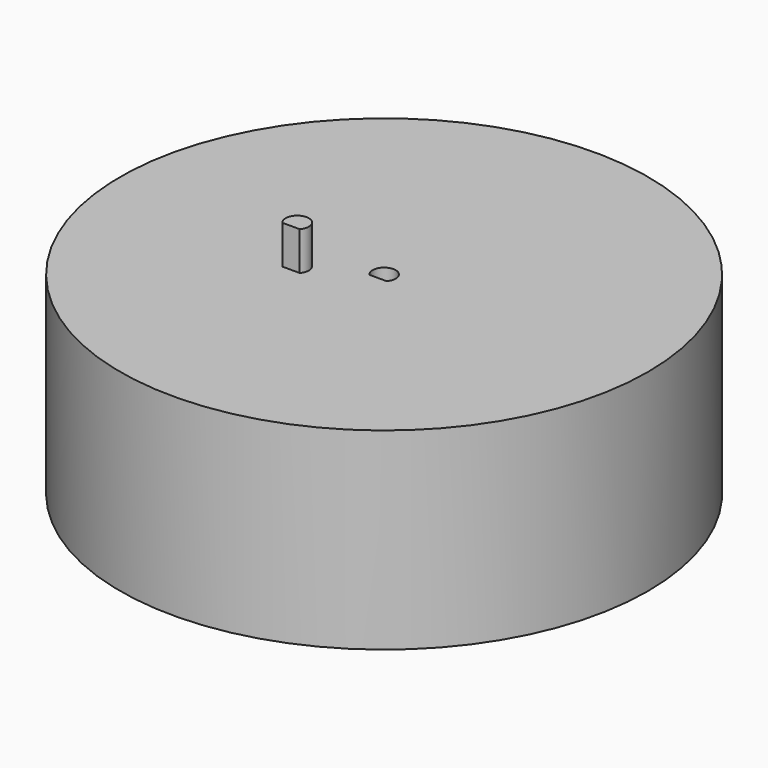
from build123d import *

# Parameters (mm, degrees)
F0_R     = 34.2051900743
F1_DEPTH = 25
F3_DEPTH = 10
F4_W     = 10
F4_H     = 7
F5_DEPTH = 20
F7_DEPTH = 10


with BuildPart() as f1:
    # F0 (on Top) → F1 (new body)
    with BuildSketch(Plane.XY):
        Circle(F0_R)
    extrude(amount=F1_DEPTH)

    # F2 (on face) → F3 (cut)
    with BuildSketch(Plane.XY.offset(25)):
        with BuildLine():
            Line((0, -1), (1.1180339887, -1))
            ThreePointArc((1.1180339887, -1), (0, 1.5), (-1.1180339887, -1))
            Line((-1.1180339887, -1), (0, -1))
        make_face()
    extrude(amount=-F3_DEPTH, mode=Mode.SUBTRACT)


with BuildPart() as f5:
    # F4 (on Top) → F5 (new body)
    with BuildSketch(Plane.XY):
        with Locations((-7.8889451153, -4.0067454018)):
            Rectangle(F4_W, F4_H)
        with BuildLine():
            Line((-12.8889451153, -0.5067454018), (-2.8889451153, -0.5067454018))
            ThreePointArc((-2.8889451153, -0.5067454018), (-7.8889451153, 2.2227708057), (-12.8889451153, -0.5067454018))
        make_face()
        with BuildLine():
            ThreePointArc((-12.8889451153, -7.5067454018), (-7.8889451153, -9.9842291943), (-2.8889451153, -7.5067454018))
            Line((-2.8889451153, -7.5067454018), (-12.8889451153, -7.5067454018))
        make_face()
    extrude(amount=F5_DEPTH)

    # F6 (on face) → F7 (join)
    with BuildSketch(Plane.XY.offset(20)):
        with BuildLine():
            Line((-7.9751741141, -5.0994232297), (-6.8571401254, -5.0994232297))
            ThreePointArc((-6.8571401254, -5.0994232297), (-7.9751741141, -2.5994232297), (-9.0932081029, -5.0994232297))
            Line((-9.0932081029, -5.0994232297), (-7.9751741141, -5.0994232297))
        make_face()
    extrude(amount=F7_DEPTH)


solid = Compound([f1.part, f5.part])
